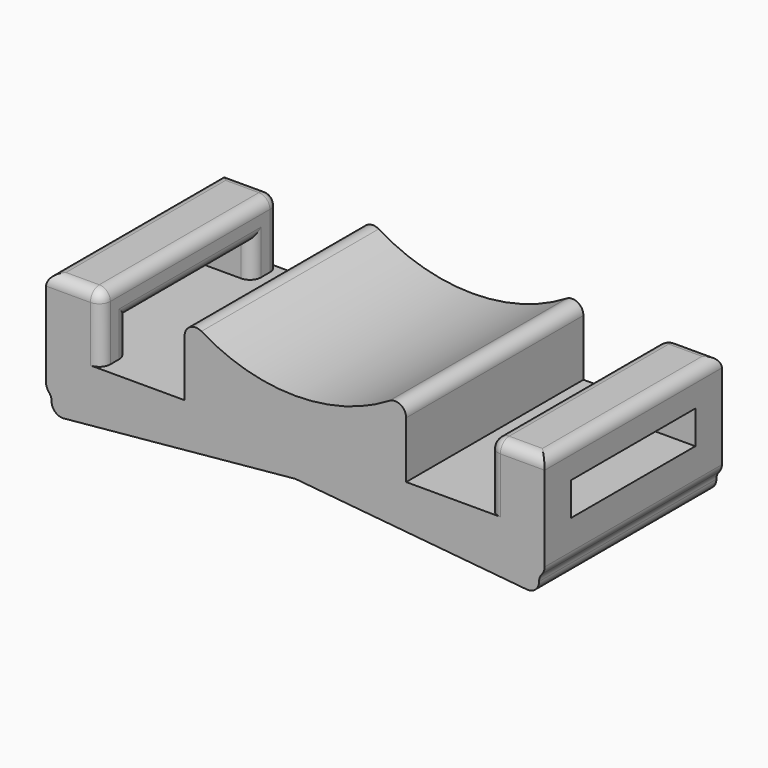
from build123d import *

# Parameters (mm, degrees)
F0_W      = 50
F0_H      = 20
F1_DEPTH  = 3
F3_DEPTH  = 10
F4_DEPTH  = 10
F5_W      = 2.5
F5_H      = 20
F5_W_2    = 5
F6_DEPTH  = 6
F7_W      = 14
F7_H      = 3
F8_DEPTH  = 25
F9_W      = 14
F9_H      = 3
F10_DEPTH = 25
F12_DEPTH = 10
F13_DEPTH = 10
F14_R     = 0.99999
F15_R     = 1
F16_W     = 2.5
F16_H     = 20
F17_DEPTH = 25
F18_W     = 2.5
F18_H     = 20
F19_DEPTH = 25
F20_R     = 0.99999


# Not quite as in the source:
# - a fillet or chamfer is up to 0.001 mm smaller than in the source, because OpenCascade refuses the exact size


with BuildPart() as f1:
    # F0 (on Top) → F1 (new body)
    with BuildSketch(Plane.XY):
        Rectangle(F0_W, F0_H)
    extrude(amount=F1_DEPTH)

    # F2 (on Front) → F3 (join)
    with BuildSketch(Plane.XZ):
        Polygon((0, 0), (-22, 0), (-22, -2.1), align=None)
        Polygon((22, 0), (0, 0), (22, -2.1), align=None)
    extrude(amount=F3_DEPTH)

    # F4 (add): faces of the model
    f4_faces = [f1.faces().sort_by_distance(p)[0] for p in [
        (14.6666666667, 0, -0.7),
        (-14.6666666667, 0, -0.7),
    ]]
    extrude(f4_faces, amount=F4_DEPTH)

    # F5 (on face) → F6 (join)
    with BuildSketch(Plane.XY.offset(3)):
        with Locations((-23.75, 0)):
            Rectangle(F5_W, F5_H)
        with Locations((-20, 0)):
            Rectangle(F5_W_2, F5_H)
        with Locations((23.75, 0)):
            Rectangle(F5_W, F5_H)
        with Locations((20, 0)):
            Rectangle(F5_W_2, F5_H)
    extrude(amount=F6_DEPTH)

    # F7 (on face) → F8 (cut)
    with BuildSketch(Plane.YZ.offset(-17.5)):
        with Locations((0, 4.5)):
            Rectangle(F7_W, F7_H)
    extrude(amount=-F8_DEPTH, mode=Mode.SUBTRACT)

    # F9 (on face) → F10 (cut)
    with BuildSketch(Plane(origin=(17.5, 0, 0), x_dir=(0, -1, 0), z_dir=(-1, 0, 0))):
        with Locations((0, 4.5)):
            Rectangle(F9_W, F9_H)
    extrude(amount=-F10_DEPTH, mode=Mode.SUBTRACT)

    # F11 (on Front) → F12 (join)
    with BuildSketch(Plane.XZ):
        with BuildLine():
            Line((-10, 10), (-10, 3))
            Line((-10, 3), (10, 3))
            Line((10, 3), (10, 10))
            ThreePointArc((10, 10), (0, 6.5968126209), (-10, 10))
        make_face()
    extrude(amount=F12_DEPTH)

    # F13 (add): a face of the model
    f13_faces = [f1.faces().sort_by_distance(p)[0] for p in [
        (0, 0, 5.4458216504),
    ]]
    extrude(f13_faces, amount=F13_DEPTH)

    # F14 (radius 1 in the source; OpenCascade refuses exactly that, so slightly less here)
    f14_edges = [f1.edges().sort_by_distance(p)[0] for p in [
        (-17.5, 0, 9),
        (-25, 0, 0),
        (-22, 0, 0),
        (-22, 0, -2.1),
        (25, 0, 0),
        (22, 0, 0),
        (22, 0, -2.1),
        (17.5, 0, 9),
        (17.5, 0, 6),
        (25, 0, 6),
        (25, -7, 4.5),
        (17.5, -7, 4.5),
        (25, 7, 4.5),
        (17.5, 7, 4.5),
        (25, 0, 3),
        (-25, 0, 6),
        (-17.5, -7, 4.5),
        (-25, -7, 4.5),
        (-25, 0, 3),
        (-17.5, 0, 6),
        (-17.5, 7, 4.5),
    ]]
    fillet(f14_edges, radius=F14_R)

    # F15
    f15_edges = [f1.edges().sort_by_distance(p)[0] for p in [
        (-10, 0, 10),
        (10, 0, 10),
    ]]
    fillet(f15_edges, radius=F15_R)

    # F16 (on face) → F17 (cut)
    with BuildSketch(Plane.XY.offset(9)):
        with Locations((-23.75, 0)):
            Rectangle(F16_W, F16_H)
    extrude(amount=-F17_DEPTH, mode=Mode.SUBTRACT)

    # F18 (on face) → F19 (cut)
    with BuildSketch(Plane.XY.offset(9)):
        with Locations((23.75, 0)):
            Rectangle(F18_W, F18_H)
    extrude(amount=-F19_DEPTH, mode=Mode.SUBTRACT)

    # F20 (radius 1 in the source; OpenCascade refuses exactly that, so slightly less here)
    f20_edges = [f1.edges().sort_by_distance(p)[0] for p in [
        (-22.5, 0, -0.13397),
        (22.5, 0, -0.13397),
        (22.5, 0, 9),
        (20.499995, -10, 9),
        (20.499995, 10, 9),
        (-20.499995, 10, 9),
        (-22.5, 0, 9),
        (-20.499995, -10, 9),
    ]]
    fillet(f20_edges, radius=F20_R)


solid = f1.part
